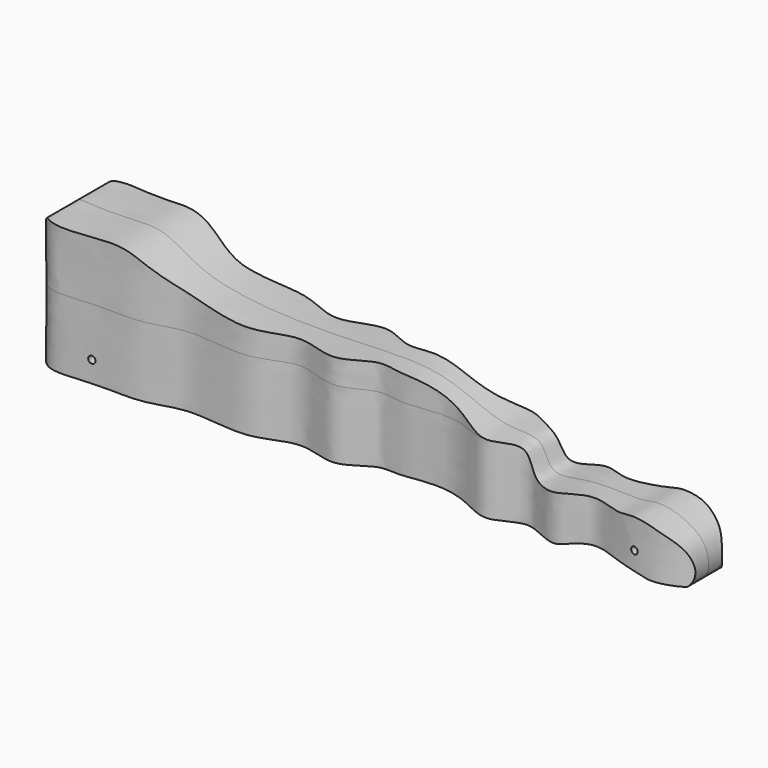
from build123d import *

# Parameters (mm, degrees)
F4_DEPTH = 22.225
F5_DEPTH = 31.75
F6_START = -88.9
F2_R     = 9.525
F6_DEPTH = 63.5
F3_R     = 1.5875
F7_DEPTH = 25.4


with BuildPart() as f4:
    # F0 (on Front) → F4 (new body, symmetric)
    with BuildSketch(Plane.XZ):
        with BuildLine():
            add(Edge.make_bspline(
                [(-142.9670453072, -32.5965434313), (-144.8278243871, -30.3883613932), (-142.241385733, -14.7737244761), (-143.1422648519, 10.1395026751), (-144.5959337062, 27.2846574857), (-138.4037672133, 26.8124108167), (-121.5635191998, 26.0038182556), (-102.4391631428, 28.6779777645), (-83.4587208601, 11.4772067647), (-23.3619462272, 9.7405110709), (17.1878006171, 13.3681745373), (37.9459718134, 4.7398039275), (52.5237597808, -1.2807508282), (68.8396351445, 0.8616085144), (71.1012115918, -14.8623372735), (90.1744070051, -8.511532739), (111.9674671254, -10.8870287554), (119.4198603819, -8.3572929445), (127.9493917953, -9.5402721156), (134.3074844591, -12.3470552792), (143.1907541752, -17.5626317129), (144.9710100765, -36.862513894), (119.2600081839, -28.7546243253), (92.262944709, -28.4748920138), (85.137266822, -32.3176394302), (67.0703247414, -31.0528913286), (56.0618729841, -32.07827397), (25.2474527833, -28.4348355831), (10.6138429564, -29.3034227223), (-15.8474975121, -31.4776092857), (-51.7125892825, -32.0859356145), (-69.2109578718, -32.5677436552), (-91.897265652, -31.8060363601), (-105.9991332313, -32.8429444293), (-122.0085335973, -32.4034071064), (-135.8881951327, -33.0401611276), (-141.7948591514, -33.98757391), (-142.9670453072, -32.5965434313)],
                knots=[0, 0, 0, 0, 0.0274041034, 0.064222771, 0.0899286626, 0.1035739681, 0.1318042592, 0.161226371, 0.1942004008, 0.2472041834, 0.2916994919, 0.3230686397, 0.3504428109, 0.3758426622, 0.3979847301, 0.4261939501, 0.4587374165, 0.4777700529, 0.4970929421, 0.5152821975, 0.5369620522, 0.5610918595, 0.5931033883, 0.6291588848, 0.6486895797, 0.6764700394, 0.7008778088, 0.7382253538, 0.7652131197, 0.8003852857, 0.8415937007, 0.8710118961, 0.9030248575, 0.929169696, 0.9565830968, 0.9827369563, 1, 1, 1, 1], degree=3))
        make_face()
    extrude(amount=F4_DEPTH, both=True)

    # F1 (on Top) → F5 (intersect, symmetric)
    with BuildSketch(Plane.XY):
        with BuildLine():
            add(Edge.make_bspline(
                [(-146.05, 0), (-146.9243635661, 4.450984412), (-147.426559273, 12.4385701998), (-140.9883503688, 20.3829688909), (-129.6241467534, 20.2914458243), (-115.7686171524, 18.7290887854), (-96.8825374889, 20.2450271437), (-80.56723806, 12.0121289678), (-51.8498741783, 19.5029786953), (-34.0373952911, 6.2420623848), (-14.5892213422, 18.2191528501), (-0.1953482778, 6.3593784856), (11.5674878205, 10.9029185725), (29.9840540179, 6.8939066418), (42.3455767563, 9.9718911723), (54.0344678577, 16.0722842939), (67.7849668703, 3.9713265354), (83.8981719567, 17.0231779396), (96.9720483384, 7.5457247281), (108.8955746266, 11.5580876019), (116.7789263398, 13.5962810955), (127.7978301262, 14.0042305545), (132.8726629181, 13.5687155003), (144.1639160089, 9.4623683765), (145.4324702953, 3.067189078), (146.05, 0)],
                knots=[0, 0, 0, 0, 0.0415608257, 0.076308925, 0.1145315433, 0.1593150234, 0.2098412934, 0.2597933207, 0.3220658438, 0.3747129059, 0.4263965483, 0.4730607233, 0.5134408275, 0.563970851, 0.6064498095, 0.6466161695, 0.6922244593, 0.7408459162, 0.7849289269, 0.8250299797, 0.8597771108, 0.8979166525, 0.9257050228, 0.9643350375, 1, 1, 1, 1], degree=3))
            add(Edge.make_bspline(
                [(-146.05, 0), (-146.9243635661, -4.450984412), (-147.426559273, -12.4385701998), (-140.9883503688, -20.3829688909), (-129.6241467534, -20.2914458243), (-115.7686171524, -18.7290887854), (-96.8825374889, -20.2450271437), (-80.56723806, -12.0121289678), (-51.8498741783, -19.5029786953), (-34.0373952911, -6.2420623848), (-14.5892213422, -18.2191528501), (-0.1953482778, -6.3593784856), (11.5674878205, -10.9029185725), (29.9840540179, -6.8939066418), (42.3455767563, -9.9718911723), (54.0344678577, -16.0722842939), (67.7849668703, -3.9713265354), (83.8981719567, -17.0231779396), (96.9720483384, -7.5457247281), (108.8955746266, -11.5580876019), (116.7789263398, -13.5962810955), (127.7978301262, -14.0042305545), (132.8726629181, -13.5687155003), (144.1639160089, -9.4623683765), (145.4324702953, -3.067189078), (146.05, 0)],
                knots=[0, 0, 0, 0, 0.0415608257, 0.076308925, 0.1145315433, 0.1593150234, 0.2098412934, 0.2597933207, 0.3220658438, 0.3747129059, 0.4263965483, 0.4730607233, 0.5134408275, 0.563970851, 0.6064498095, 0.6466161695, 0.6922244593, 0.7408459162, 0.7849289269, 0.8250299797, 0.8597771108, 0.8979166525, 0.9257050228, 0.9643350375, 1, 1, 1, 1], degree=3))
        make_face()
    extrude(amount=F5_DEPTH, both=True, mode=Mode.INTERSECT)

    # F2 (on Right) → F6 (cut)
    with BuildSketch(Plane.YZ.offset(F6_START)):
        Circle(F2_R)
    extrude(amount=-F6_DEPTH, mode=Mode.SUBTRACT)

    # F3 (on Front) → F7 (cut, symmetric)
    with BuildSketch(Plane.XZ):
        with Locations((-120.65, -22.225)):
            Circle(F3_R)
        with Locations((120.65, -22.225)):
            Circle(F3_R)
    extrude(amount=F7_DEPTH, both=True, mode=Mode.SUBTRACT)


solid = f4.part
